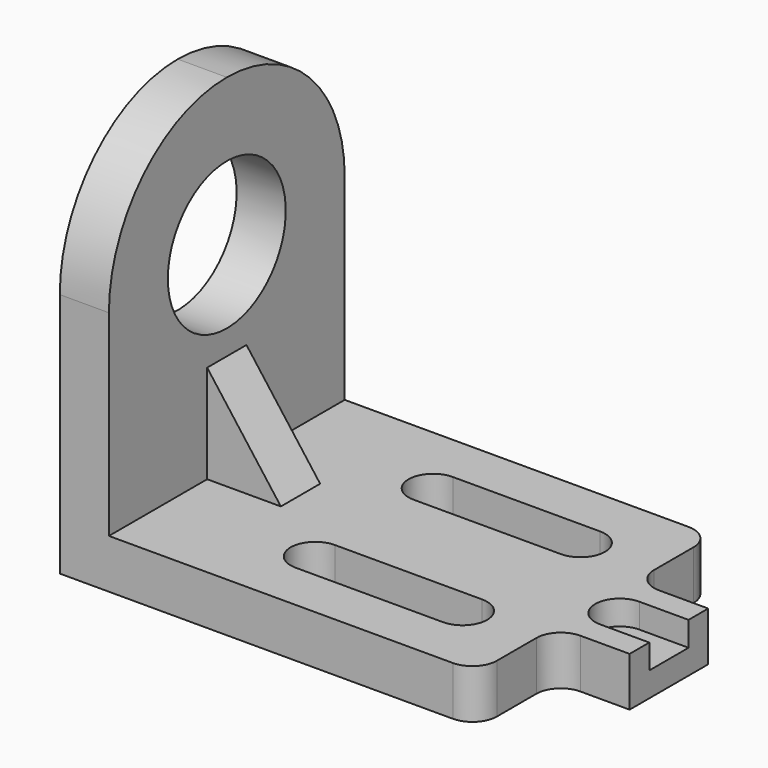
from build123d import *

# Parameters (mm, degrees)
F1_DEPTH = 203.2
F2_DEPTH = 25.4
F3_DEPTH = 12.7
F0_W     = 38.1
F0_H     = 25.4
F4_DEPTH = 76.2
F6_R     = 76.19999
F7_D     = 76.2
F8_SIZE2 = 38.09999
F8_SIZE  = 50.79999


# Not quite as in the source:
# - a fillet or chamfer is up to 0.001 mm smaller than in the source, because OpenCascade refuses the exact size


with BuildPart() as f1:
    # F0 (on Top) → F1 (new body)
    with BuildSketch(Plane.XY):
        Polygon((25.4, 0), (0, 0), (0, -152.4), (25.4, -152.4), (25.4, -88.9), (25.4, -63.5), align=None)
    extrude(amount=F1_DEPTH)

    # F0 (on Top) → F2 (join)
    with BuildSketch(Plane.XY):
        with BuildLine():
            Line((101.6, 0), (25.4, 0))
            Line((25.4, 0), (25.4, -63.5))
            Line((25.4, -63.5), (63.5, -63.5))
            Line((63.5, -63.5), (63.5, -88.9))
            Line((63.5, -88.9), (25.4, -88.9))
            Line((25.4, -88.9), (25.4, -152.4))
            Line((25.4, -152.4), (101.6, -152.4))
            Line((101.6, -152.4), (203.2, -152.4))
            ThreePointArc((203.2, -152.4), (212.1802561211, -148.6802561211), (215.9, -139.7))
            Line((215.9, -139.7), (215.9, -114.3))
            ThreePointArc((215.9, -114.3), (219.6197438789, -105.3197438789), (228.6, -101.6))
            Line((228.6, -101.6), (254, -101.6))
            Line((254, -101.6), (254, -88.9))
            Line((254, -88.9), (228.6, -88.9))
            ThreePointArc((228.6, -88.9), (215.9, -76.2), (228.6, -63.5))
            Line((228.6, -63.5), (254, -63.5))
            Line((254, -63.5), (254, -50.8))
            Line((254, -50.8), (228.6, -50.8))
            ThreePointArc((228.6, -50.8), (219.6197438789, -47.0802561211), (215.9, -38.1))
            Line((215.9, -38.1), (215.9, -12.7))
            ThreePointArc((215.9, -12.7), (212.1802561211, -3.7197438789), (203.2, 0))
            Line((203.2, 0), (101.6, 0))
        make_face()
        with BuildLine():
            Line((177.8, -127), (101.6, -127))
            ThreePointArc((101.6, -127), (88.9, -114.3), (101.6, -101.6))
            Line((101.6, -101.6), (177.8, -101.6))
            ThreePointArc((177.8, -101.6), (190.5, -114.3), (177.8, -127))
        make_face(mode=Mode.SUBTRACT)
        with BuildLine():
            ThreePointArc((101.6, -50.8), (88.9, -38.1), (101.6, -25.4))
            Line((101.6, -25.4), (177.8, -25.4))
            ThreePointArc((177.8, -25.4), (190.5, -38.1), (177.8, -50.8))
            Line((177.8, -50.8), (101.6, -50.8))
        make_face(mode=Mode.SUBTRACT)
    extrude(amount=F2_DEPTH)

    # F0 (on Top) → F3 (join)
    with BuildSketch(Plane.XY):
        Polygon((254, -88.9), (254, -63.5), (228.6, -63.5), (228.6, -76.2), (228.6, -88.9), align=None)
        with BuildLine():
            Line((228.6, -76.2), (228.6, -63.5))
            ThreePointArc((228.6, -63.5), (215.9, -76.2), (228.6, -88.9))
            Line((228.6, -88.9), (228.6, -76.2))
        make_face()
    extrude(amount=F3_DEPTH)

    # F0 (on Top) → F4 (join)
    with BuildSketch(Plane.XY):
        with Locations((44.45, -76.2)):
            Rectangle(F0_W, F0_H)
    extrude(amount=F4_DEPTH)

    # F6 (radius 76.2 in the source; OpenCascade refuses exactly that, so slightly less here)
    f6_edges = [f1.edges().sort_by_distance(p)[0] for p in [
        (12.7, -152.4, 203.2),
        (12.7, 0, 203.2),
    ]]
    fillet(f6_edges, radius=F6_R)

    # F7 (through all)
    with Locations(Plane(origin=(0, 0, 0), x_dir=(0, 1, 0), z_dir=(-1, 0, 0))):
        with Locations((-76.2, -127)):
            Hole(F7_D / 2)

    # F8 (size 50.8 and 38.0999999365 in the source; OpenCascade refuses exactly that, so slightly less here)
    f8_edges = [f1.edges().sort_by_distance(p)[0] for p in [
        (63.5, -76.2, 76.2),
    ]]
    f8_side = f1.faces().sort_by_distance((63.5, -76.2, 50.8))[0]
    chamfer(f8_edges, length=F8_SIZE, length2=F8_SIZE2, reference=f8_side)


solid = f1.part
